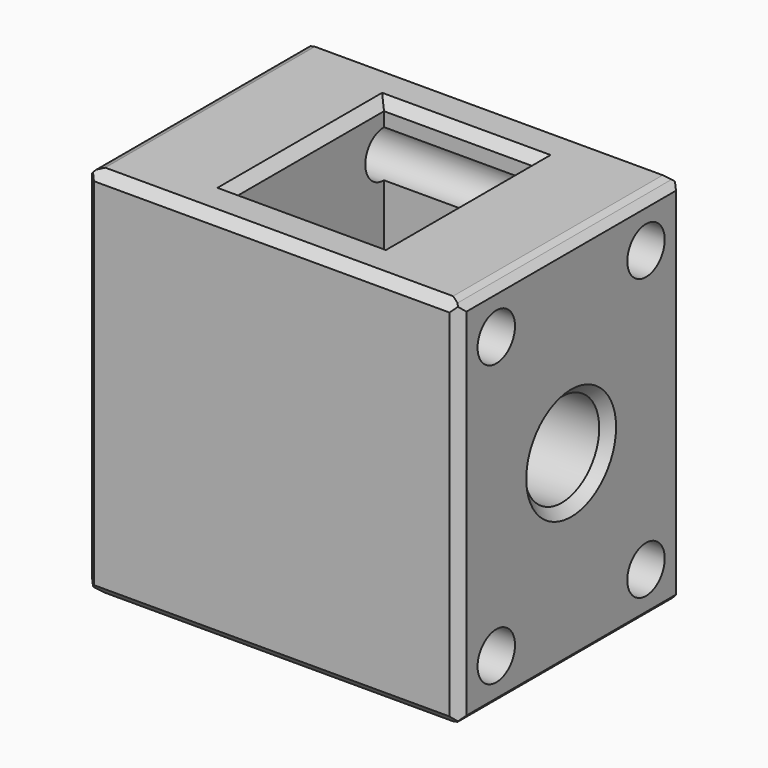
from build123d import *

# Parameters (mm, degrees)
F0_W         = 150
F0_H         = 200
F0_R         = 25
F1_DEPTH     = 200
F2_SIZE      = 5
F3_R         = 12.5
F4_DEPTH     = 200.001
F5_W         = 80
F5_H         = 100
F6_DEPTH     = 200.001
F7_T1_DEPTH  = 215.7168298797
F7_T3_DEPTH  = 161.2857086021
F7_T5_DEPTH  = 100
F7_T7_DEPTH  = 80
F7_T13_DEPTH = 112.8584149398
F7_T17_DEPTH = 92.8584149398
F7_T24_DEPTH = 112.8584149398
F7_T28_DEPTH = 92.8584149398
F7_T35_DEPTH = 92.8584149398
F7_T39_DEPTH = 112.8584149398
F7_T46_DEPTH = 112.8584149398
F7_T50_DEPTH = 92.8584149398
F7_T57_DEPTH = 112.8584149398
F7_T61_DEPTH = 92.8584149398
F7_T68_DEPTH = 112.8584149398
F7_T72_DEPTH = 92.8584149398
F7_T79_DEPTH = 112.8584149398
F7_T83_DEPTH = 92.8584149398
F7_T90_DEPTH = 112.8584149398
F7_T94_DEPTH = 92.8584149398


# Not quite as in the source:
# - a fillet or chamfer that OpenCascade refuses, or shapes differently, is made with other operations: its cross-section is extruded or revolved along the edge and cut away or added


with BuildPart() as f1:
    # F0 (on Right) → F1 (new body)
    with BuildSketch(Plane.YZ):
        Rectangle(F0_W, F0_H)
        Circle(F0_R, mode=Mode.SUBTRACT)
    extrude(amount=-F1_DEPTH)

    # F2
    f2_edges = [f1.edges().sort_by_distance(p)[0] for p in [
        (0, 0, -100),
        (0, 75, 0),
        (0, 0, 100),
        (0, -75, 0),
        (0, -25, 0),
        (-200, 0, -100),
        (-200, 75, 0),
        (-200, 0, 100),
        (-200, -75, 0),
        (-200, -25, 0),
    ]]
    chamfer(f2_edges, length=F2_SIZE)

    # F3 (on face) → F4 (cut, through all)
    with BuildSketch(Plane(origin=(-200, 0, 0), x_dir=(0, -1, 0), z_dir=(-1, 0, 0))):
        with Locations((-50, -75)):
            Circle(F3_R)
        with Locations((-50, 75)):
            Circle(F3_R)
        with Locations((50, -75)):
            Circle(F3_R)
        with Locations((50, 75)):
            Circle(F3_R)
    extrude(amount=-F4_DEPTH, mode=Mode.SUBTRACT)

    # F5 (on face) → F6 (cut, through all)
    with BuildSketch(Plane(origin=(0, 0, -100), x_dir=(1, 0, 0), z_dir=(0, 0, -1))):
        with Locations((-100, 0)):
            Rectangle(F5_W, F5_H)
    extrude(amount=-F6_DEPTH, mode=Mode.SUBTRACT)

    # F7: chamfer of 5 on 16 edges, made by hand

    # F7_s2 → F7_t1 (cut)
    with BuildSketch(Plane.YZ.offset(-207.8584149398)):
        Polygon((-70, -100), (-75, -95), (-75, -100), align=None)
        Polygon((70, -100), (75, -95), (75, -100), align=None)
        Polygon((75, 95), (70, 100), (75, 100), align=None)
        Polygon((-75, 95), (-70, 100), (-75, 100), align=None)
    extrude(amount=F7_T1_DEPTH, mode=Mode.SUBTRACT)

    # F7_s4 → F7_t3 (cut)
    with BuildSketch(Plane.XZ.offset(-80.6428543011)):
        Polygon((-7.0710678119, -100), (-3.5355339059, -98.5355339059), (-5, -100), align=None)
        Polygon((-192.9289321881, -100), (-196.4644660941, -98.5355339059), (-195, -100), align=None)
        Polygon((-7.0710678119, 100), (-3.5355339059, 98.5355339059), (-5, 100), align=None)
        Polygon((-192.9289321881, 100), (-196.4644660941, 98.5355339059), (-195, 100), align=None)
    extrude(amount=F7_T3_DEPTH, mode=Mode.SUBTRACT)

    # F7_s6 → F7_t5 (cut)
    with BuildSketch(Plane.XZ.offset(-50)):
        Polygon((-55, -100), (-60, -95), (-60, -100), align=None)
        Polygon((-145, -100), (-140, -95), (-140, -100), align=None)
        Polygon((-60, 95), (-55, 100), (-60, 100), align=None)
        Polygon((-140, 95), (-145, 100), (-140, 100), align=None)
    extrude(amount=F7_T5_DEPTH, mode=Mode.SUBTRACT)

    # F7_s8 → F7_t7 (cut)
    with BuildSketch(Plane.YZ.offset(-140)):
        Polygon((-55, -100), (-50, -95), (-50, -100), align=None)
        Polygon((55, -100), (50, -95), (50, -100), align=None)
        Polygon((55, 100), (50, 95), (50, 100), align=None)
        Polygon((-55, 100), (-50, 95), (-50, 100), align=None)
    extrude(amount=F7_T7_DEPTH, mode=Mode.SUBTRACT)


with BuildPart() as f7_tool11:
    # F7_s12 → F7_t13 (new body)
    with BuildSketch(Plane.XZ.offset(-62.8584149398)):
        Polygon((-55, -100), (-60, -95), (-60, -100), align=None)
    extrude(amount=F7_T13_DEPTH)

    split(bisect_by=Plane.XZ.offset(-50), keep=Keep.BOTTOM)


with BuildPart() as f7_tool15:
    # F7_s16 → F7_t17 (new body)
    with BuildSketch(Plane.YZ.offset(-140)):
        Polygon((55, -100), (50, -95), (50, -100), align=None)
    extrude(amount=F7_T17_DEPTH)

    split(bisect_by=Plane.YZ.offset(-60), keep=Keep.TOP)


with BuildPart() as f7_tool11_1:
    add(f7_tool11.part)

    # F7_t19: intersect F7_tool15
    add(f7_tool15.part, mode=Mode.INTERSECT)


with BuildPart() as f1_1:
    add(f1.part)

    # F7_t9: cut F7_tool11
    add(f7_tool11_1.part, mode=Mode.SUBTRACT)


with BuildPart() as f7_tool22:
    # F7_s23 → F7_t24 (new body)
    with BuildSketch(Plane.XZ.offset(-50)):
        Polygon((-55, -100), (-60, -95), (-60, -100), align=None)
    extrude(amount=F7_T24_DEPTH)

    split(bisect_by=Plane.XZ.offset(50), keep=Keep.TOP)


with BuildPart() as f7_tool26:
    # F7_s27 → F7_t28 (new body)
    with BuildSketch(Plane.YZ.offset(-47.1415850602)):
        Polygon((-55, -100), (-50, -95), (-50, -100), align=None)
    extrude(amount=-F7_T28_DEPTH)

    split(bisect_by=Plane.YZ.offset(-60), keep=Keep.TOP)


with BuildPart() as f7_tool22_1:
    add(f7_tool22.part)

    # F7_t30: intersect F7_tool26
    add(f7_tool26.part, mode=Mode.INTERSECT)


with BuildPart() as f1_2:
    add(f1_1.part)

    # F7_t20: cut F7_tool22
    add(f7_tool22_1.part, mode=Mode.SUBTRACT)


with BuildPart() as f7_tool33:
    # F7_s34 → F7_t35 (new body)
    with BuildSketch(Plane.YZ.offset(-60)):
        Polygon((-55, -100), (-50, -95), (-50, -100), align=None)
    extrude(amount=-F7_T35_DEPTH)

    split(bisect_by=Plane.YZ.offset(-140), keep=Keep.BOTTOM)


with BuildPart() as f7_tool37:
    # F7_s38 → F7_t39 (new body)
    with BuildSketch(Plane.XZ.offset(62.8584149398)):
        Polygon((-145, -100), (-140, -95), (-140, -100), align=None)
    extrude(amount=-F7_T39_DEPTH)

    split(bisect_by=Plane.XZ.offset(50), keep=Keep.TOP)


with BuildPart() as f7_tool33_1:
    add(f7_tool33.part)

    # F7_t41: intersect F7_tool37
    add(f7_tool37.part, mode=Mode.INTERSECT)


with BuildPart() as f1_3:
    add(f1_2.part)

    # F7_t31: cut F7_tool33
    add(f7_tool33_1.part, mode=Mode.SUBTRACT)


with BuildPart() as f7_tool44:
    # F7_s45 → F7_t46 (new body)
    with BuildSketch(Plane.XZ.offset(50)):
        Polygon((-145, -100), (-140, -95), (-140, -100), align=None)
    extrude(amount=-F7_T46_DEPTH)

    split(bisect_by=Plane.XZ.offset(-50), keep=Keep.BOTTOM)


with BuildPart() as f7_tool48:
    # F7_s49 → F7_t50 (new body)
    with BuildSketch(Plane.YZ.offset(-152.8584149398)):
        Polygon((55, -100), (50, -95), (50, -100), align=None)
    extrude(amount=F7_T50_DEPTH)

    split(bisect_by=Plane.YZ.offset(-140), keep=Keep.BOTTOM)


with BuildPart() as f7_tool44_1:
    add(f7_tool44.part)

    # F7_t52: intersect F7_tool48
    add(f7_tool48.part, mode=Mode.INTERSECT)


with BuildPart() as f1_4:
    add(f1_3.part)

    # F7_t42: cut F7_tool44
    add(f7_tool44_1.part, mode=Mode.SUBTRACT)


with BuildPart() as f7_tool55:
    # F7_s56 → F7_t57 (new body)
    with BuildSketch(Plane.XZ.offset(62.8584149398)):
        Polygon((-60, 95), (-55, 100), (-60, 100), align=None)
    extrude(amount=-F7_T57_DEPTH)

    split(bisect_by=Plane.XZ.offset(50), keep=Keep.TOP)


with BuildPart() as f7_tool59:
    # F7_s60 → F7_t61 (new body)
    with BuildSketch(Plane.YZ.offset(-140)):
        Polygon((-55, 100), (-50, 95), (-50, 100), align=None)
    extrude(amount=F7_T61_DEPTH)

    split(bisect_by=Plane.YZ.offset(-60), keep=Keep.TOP)


with BuildPart() as f7_tool55_1:
    add(f7_tool55.part)

    # F7_t63: intersect F7_tool59
    add(f7_tool59.part, mode=Mode.INTERSECT)


with BuildPart() as f1_5:
    add(f1_4.part)

    # F7_t53: cut F7_tool55
    add(f7_tool55_1.part, mode=Mode.SUBTRACT)


with BuildPart() as f7_tool66:
    # F7_s67 → F7_t68 (new body)
    with BuildSketch(Plane.XZ.offset(50)):
        Polygon((-60, 95), (-55, 100), (-60, 100), align=None)
    extrude(amount=-F7_T68_DEPTH)

    split(bisect_by=Plane.XZ.offset(-50), keep=Keep.BOTTOM)


with BuildPart() as f7_tool70:
    # F7_s71 → F7_t72 (new body)
    with BuildSketch(Plane.YZ.offset(-47.1415850602)):
        Polygon((55, 100), (50, 95), (50, 100), align=None)
    extrude(amount=-F7_T72_DEPTH)

    split(bisect_by=Plane.YZ.offset(-60), keep=Keep.TOP)


with BuildPart() as f7_tool66_1:
    add(f7_tool66.part)

    # F7_t74: intersect F7_tool70
    add(f7_tool70.part, mode=Mode.INTERSECT)


with BuildPart() as f1_6:
    add(f1_5.part)

    # F7_t64: cut F7_tool66
    add(f7_tool66_1.part, mode=Mode.SUBTRACT)


with BuildPart() as f7_tool77:
    # F7_s78 → F7_t79 (new body)
    with BuildSketch(Plane.XZ.offset(-62.8584149398)):
        Polygon((-140, 95), (-145, 100), (-140, 100), align=None)
    extrude(amount=F7_T79_DEPTH)

    split(bisect_by=Plane.XZ.offset(-50), keep=Keep.BOTTOM)


with BuildPart() as f7_tool81:
    # F7_s82 → F7_t83 (new body)
    with BuildSketch(Plane.YZ.offset(-60)):
        Polygon((55, 100), (50, 95), (50, 100), align=None)
    extrude(amount=-F7_T83_DEPTH)

    split(bisect_by=Plane.YZ.offset(-140), keep=Keep.BOTTOM)


with BuildPart() as f7_tool77_1:
    add(f7_tool77.part)

    # F7_t85: intersect F7_tool81
    add(f7_tool81.part, mode=Mode.INTERSECT)


with BuildPart() as f1_7:
    add(f1_6.part)

    # F7_t75: cut F7_tool77
    add(f7_tool77_1.part, mode=Mode.SUBTRACT)


with BuildPart() as f7_tool88:
    # F7_s89 → F7_t90 (new body)
    with BuildSketch(Plane.XZ.offset(-50)):
        Polygon((-140, 95), (-145, 100), (-140, 100), align=None)
    extrude(amount=F7_T90_DEPTH)

    split(bisect_by=Plane.XZ.offset(50), keep=Keep.TOP)


with BuildPart() as f7_tool92:
    # F7_s93 → F7_t94 (new body)
    with BuildSketch(Plane.YZ.offset(-152.8584149398)):
        Polygon((-55, 100), (-50, 95), (-50, 100), align=None)
    extrude(amount=F7_T94_DEPTH)

    split(bisect_by=Plane.YZ.offset(-140), keep=Keep.BOTTOM)


with BuildPart() as f7_tool88_1:
    add(f7_tool88.part)

    # F7_t96: intersect F7_tool92
    add(f7_tool92.part, mode=Mode.INTERSECT)


with BuildPart() as f1_8:
    add(f1_7.part)

    # F7_t86: cut F7_tool88
    add(f7_tool88_1.part, mode=Mode.SUBTRACT)


solid = f1_8.part
